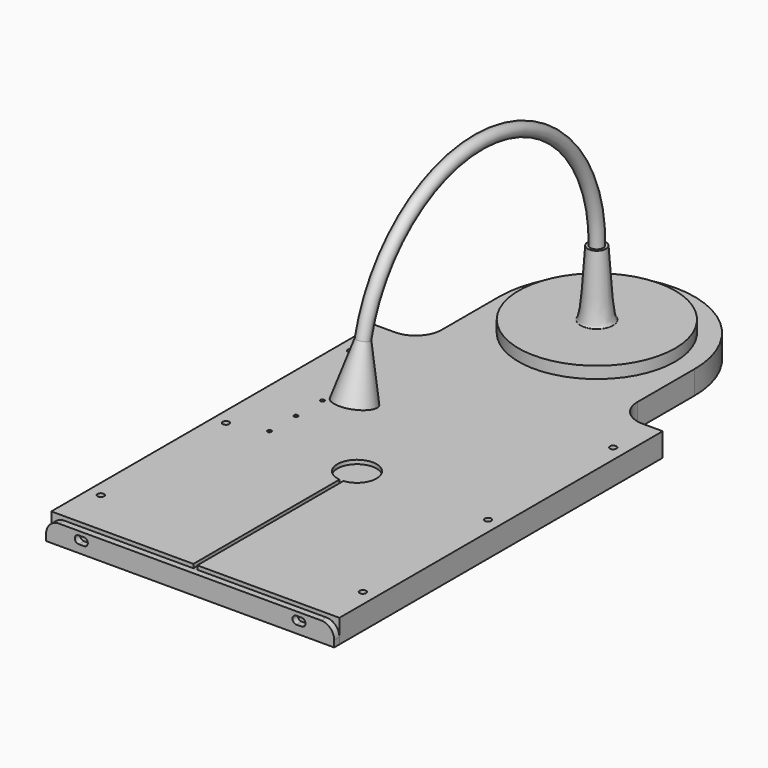
from build123d import *

# Parameters (mm, degrees)
F0_R       = 2.5
F1_DEPTH   = 18
F2_R       = 1.5
F3_DEPTH   = 1
F2_R_2     = 60
F4_DEPTH   = 3
F6_DEPTH   = 5
F10_R      = 5
F15_R      = 15
F13_FACE_R = 5
F17_R      = 7.5
F18_DEPTH  = 15


# Not quite as in the source:
# - a feature names something its author has since deleted; it is built from what else it names


with BuildPart() as f1:
    # F0 (on Top) → F1 (new body)
    with BuildSketch(Plane.XY):
        with BuildLine():
            Line((0, 310), (0, 0))
            Line((0, 0), (221, 0))
            Line((221, 0), (221, 310))
            Line((221, 310), (205.5, 310))
            ThreePointArc((205.5, 310), (191.3578643763, 315.8578643763), (185.5, 330))
            Line((185.5, 330), (185.5, 385))
            ThreePointArc((185.5, 385), (110.5, 460), (35.5, 385))
            Line((35.5, 385), (35.5, 330))
            ThreePointArc((35.5, 330), (29.6421356237, 315.8578643763), (15.5, 310))
            Line((15.5, 310), (0, 310))
        make_face()
        with Locations((10, 35)):
            Circle(F0_R, mode=Mode.SUBTRACT)
        with Locations((10, 155)):
            Circle(F0_R, mode=Mode.SUBTRACT)
        with Locations((211, 35)):
            Circle(F0_R, mode=Mode.SUBTRACT)
        with Locations((211, 155)):
            Circle(F0_R, mode=Mode.SUBTRACT)
        with Locations((10, 275)):
            Circle(F0_R, mode=Mode.SUBTRACT)
        with Locations((211, 275)):
            Circle(F0_R, mode=Mode.SUBTRACT)
    extrude(amount=F1_DEPTH)

    # F2 (on face) → F3 (cut)
    with BuildSketch(Plane.XY.offset(18)):
        with Locations((37, 162.9)):
            Circle(F2_R)
        with Locations((37, 188.3)):
            Circle(F2_R)
        with Locations((37, 213.7)):
            Circle(F2_R)
        with Locations((37, 239.1)):
            Circle(F2_R)
    extrude(amount=-F3_DEPTH, mode=Mode.SUBTRACT)

    # F2 (on face) → F4 (cut)
    with BuildSketch(Plane.XY.offset(18)):
        with BuildLine():
            Line((112, 0), (112, 140.0751884434))
            ThreePointArc((112, 140.0751884434), (110.5, 170), (109, 140.0751884434))
            Line((109, 140.0751884434), (109, 0))
            Line((109, 0), (112, 0))
        make_face()
        with Locations((110.5, 385)):
            Circle(F2_R_2)
    extrude(amount=-F4_DEPTH, mode=Mode.SUBTRACT)


with BuildPart() as f6:
    # F5 (on Front) → F6 (new body)
    with BuildSketch(Plane.XZ):
        with BuildLine():
            Line((211, 15), (10, 15))
            ThreePointArc((10, 15), (2.9289321881, 12.0710678119), (0, 5))
            Line((0, 5), (0, 0))
            Line((0, 0), (221, 0))
            Line((221, 0), (221, 5))
            ThreePointArc((221, 5), (218.0710678119, 12.0710678119), (211, 15))
        make_face()
        with BuildLine():
            ThreePointArc((25, 6), (22, 9), (25, 12))
            Line((25, 12), (29, 12))
            ThreePointArc((29, 12), (32, 9), (29, 6))
            Line((29, 6), (25, 6))
        make_face(mode=Mode.SUBTRACT)
        with BuildLine():
            Line((192, 12), (196, 12))
            ThreePointArc((196, 12), (199, 9), (196, 6))
            Line((196, 6), (192, 6))
            ThreePointArc((192, 6), (189, 9), (192, 12))
        make_face(mode=Mode.SUBTRACT)
    extrude(amount=F6_DEPTH)


with BuildPart() as f9:
    # F8 (on offset) → F9 (revolve)
    with BuildSketch(Plane.XZ.offset(-385)):
        with BuildLine():
            Line((110.5, 77), (110.5, 15))
            Line((110.5, 15), (170.5, 15))
            Line((170.5, 15), (170.5, 27))
            Line((170.5, 27), (123.0226124214, 27))
            add(Edge.make_bspline(
                [(123, 27), (123.007529237, 26.9997522408), (123.0150667195, 26.9997525006), (123.0226124214, 27)],
                knots=[0.4988200942, 0.4988200942, 0.4988200942, 0.4988200942, 0.5003949515, 0.5003949515, 0.5003949515, 0.5003949515], degree=3))
            add(Edge.make_bspline(
                [(117.5, 77), (119.0575952544, 52.0392376011), (120.6151905087, 27.0784752021), (123, 27)],
                knots=[0, 0, 0, 0, 0.4988200942, 0.4988200942, 0.4988200942, 0.4988200942], degree=3))
            Line((117.5, 77), (110.5, 77))
        make_face()
    revolve(axis=Axis((110.5, 385, 38.5), (0, 0, 1)))

    # F13: sweep along a path in F12
    with BuildLine(Plane.YZ.offset(110.5)) as f13_path:
        ThreePointArc((385, 77), (285.5138023174, 192.1246330091), (160.772137354, 105))
    # F10 (on face) → F13 (sweep)
    with BuildSketch(Plane.XY.offset(77)):
        with Locations((110.5, 385)):
            Circle(F10_R)
    sweep(path=f13_path.line)

    # F15 (on offset) → F16 section 0
    with BuildSketch(Plane(origin=(0, 19.562950875, 93.6379514405), x_dir=(1, 0, 0), z_dir=(0, -0.2045057041, -0.9788653722))):
        with Locations((110.5, -135.9011791469)):
            Circle(F15_R)
    # F13_face (on face) → F16 section 1
    with BuildSketch(Plane(origin=(110.5, 160.772137354, 105), x_dir=(1, 0, 0), z_dir=(0, -0.2045057041, -0.9788653722))):
        Circle(F13_FACE_R)
    loft()

    # F17 (on face) → F18 (cut)
    with BuildSketch(Plane(origin=(0, 19.562950875, 93.6379514405), x_dir=(1, 0, 0), z_dir=(0, -0.2045057041, -0.9788653722))):
        with Locations((110.5, -135.9011791469)):
            Circle(F17_R)
    extrude(amount=-F18_DEPTH, mode=Mode.SUBTRACT)


solid = Compound([f1.part, f6.part, f9.part])
